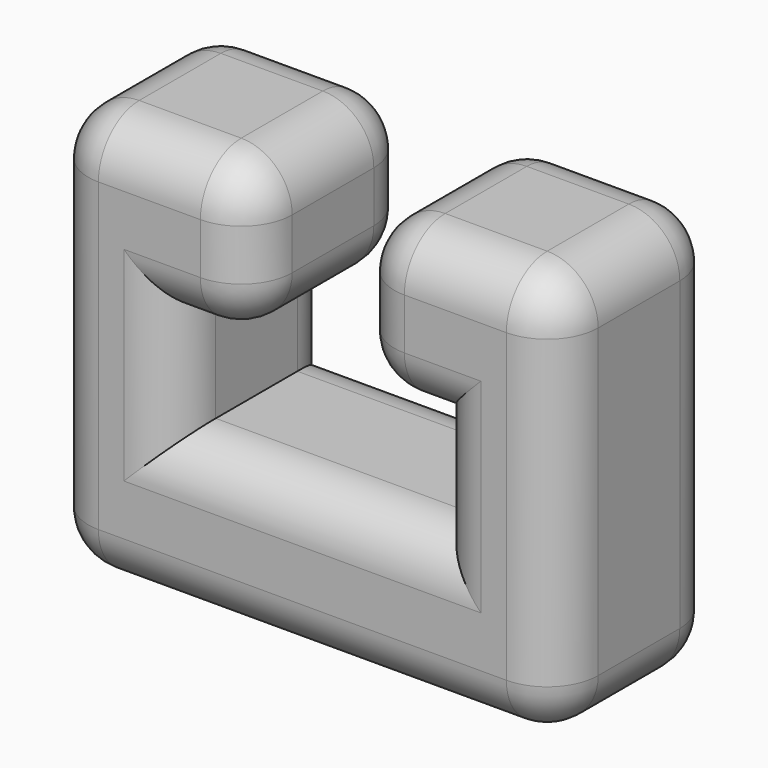
from build123d import *

# Parameters (mm, degrees)
F1_DEPTH     = 4
F2_R         = 1
F3_T1_DEPTH  = 2
F3_S5_W      = 1
F3_S5_H      = 1
F3_T6_DEPTH  = 1
F3_S11_W     = 1
F3_S11_H     = 1
F3_T12_DEPTH = 1


# Not quite as in the source:
# - a fillet or chamfer that OpenCascade refuses, or shapes differently, is made with other operations: its cross-section is extruded or revolved along the edge and cut away or added


with BuildPart() as f1:
    # F0 (on Front) → F1 (new body)
    with BuildSketch(Plane.XZ):
        Polygon((-5, 0), (0, 0), (5, 0), (5, 8), (1, 8), (1, 5), (2.5, 5), (2.5, 3), (0, 3), (-2.5, 3), (-2.5, 5), (-1, 5), (-1, 8), (-5, 8), align=None)
    extrude(amount=F1_DEPTH)

    # F2
    f2_edges = [f1.edges().sort_by_distance(p)[0] for p in [
        (3, -4, 8),
        (5, -4, 4),
        (5, -2, 8),
        (-3, -4, 8),
        (0, -4, 0),
        (1, -4, 6.5),
        (1.75, -4, 5),
        (2.5, -4, 4),
        (0, -4, 3),
        (-2.5, -4, 4),
        (-1.75, -4, 5),
        (-1, -4, 6.5),
        (-5, -4, 4),
        (-1, -2, 8),
        (-5, -2, 8),
        (-3, 0, 8),
        (-1, -2, 5),
        (-1, 0, 6.5),
        (1, -2, 8),
        (3, 0, 8),
        (5, -2, 0),
        (5, 0, 4),
        (0, 0, 0),
        (1, 0, 6.5),
        (1.75, 0, 5),
        (2.5, 0, 4),
        (0, 0, 3),
        (-2.5, 0, 4),
        (-1.75, 0, 5),
        (-5, 0, 4),
        (-5, -2, 0),
    ]]
    fillet(f2_edges, radius=F2_R)

    # F3: fillet of radius 1 on 1 edges, made by hand

    # F3_s2 → F3_t1 (cut)
    with BuildSketch(Plane.XZ.offset(1)):
        with BuildLine():
            ThreePointArc((1, 6), (1.2928932188, 5.2928932188), (2, 5))
            Line((2, 5), (1, 5))
            Line((1, 5), (1, 6))
        make_face()
    extrude(amount=F3_T1_DEPTH, mode=Mode.SUBTRACT)


with BuildPart() as f3_tool4:
    # F3_s5 → F3_t6 (new body)
    with BuildSketch(Plane.YZ.offset(2)):
        with Locations((-0.5, 5.5)):
            Rectangle(F3_S5_W, F3_S5_H)
    extrude(amount=-F3_T6_DEPTH)

    # F3_s7 → F3_t8 (revolve, cut)
    with BuildSketch(Plane(origin=(2, -1, 6), x_dir=(0, -0.7071067812, 0.7071067812), z_dir=(0, -0.7071067812, -0.7071067812))):
        with BuildLine():
            ThreePointArc((0, -1), (1, 0), (0, 1))
            Line((0, 1), (0, -1))
        make_face()
    revolve(axis=Axis((2, -1, 6), (-1, 0, 0)), mode=Mode.SUBTRACT)


with BuildPart() as f1_1:
    add(f1.part)

    # F3_t3: cut F3_tool4
    add(f3_tool4.part, mode=Mode.SUBTRACT)


with BuildPart() as f3_tool10:
    # F3_s11 → F3_t12 (new body)
    with BuildSketch(Plane.YZ.offset(2)):
        with Locations((-3.5, 5.5)):
            Rectangle(F3_S11_W, F3_S11_H)
    extrude(amount=-F3_T12_DEPTH)

    # F3_s13 → F3_t14 (revolve, cut)
    with BuildSketch(Plane(origin=(2, -3, 6), x_dir=(0, 0.7071067812, 0.7071067812), z_dir=(0, -0.7071067812, 0.7071067812))):
        with BuildLine():
            ThreePointArc((0, -1), (1, 0), (0, 1))
            Line((0, 1), (0, -1))
        make_face()
    revolve(axis=Axis((2, -3, 6), (-1, 0, 0)), mode=Mode.SUBTRACT)


with BuildPart() as f1_2:
    add(f1_1.part)

    # F3_t9: cut F3_tool10
    add(f3_tool10.part, mode=Mode.SUBTRACT)


solid = f1_2.part
